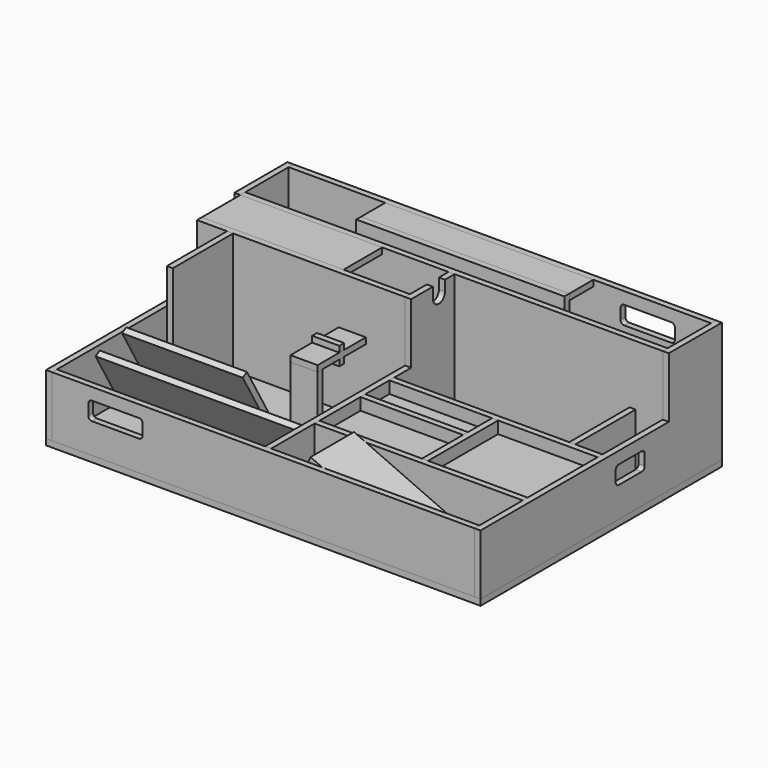
from build123d import *

# Parameters (mm, degrees)
F0_W      = 720
F0_H      = 500
F1_DEPTH  = 10
F3_DEPTH  = 10
F5_DEPTH  = 10
F6_W      = 700
F6_H      = 100
F7_DEPTH  = 10
F8_W      = 700
F8_H      = 200
F9_DEPTH  = 10
F11_DEPTH = 10
F12_W     = 345
F12_H     = 50
F13_DEPTH = 10
F14_W     = 345
F14_H     = 200
F15_DEPTH = 10
F16_W     = 235
F16_H     = 80
F17_DEPTH = 10
F19_DEPTH = 10
F21_DEPTH = 10
F22_W     = 10
F22_H     = 100
F23_DEPTH = 345
F24_W     = 10
F24_H     = 100
F25_DEPTH = 125
F26_W     = 145
F26_H     = 10
F27_DEPTH = 170
F28_W     = 145
F28_H     = 100
F29_DEPTH = 10
F30_W     = 170
F30_H     = 10
F31_DEPTH = 20
F32_W     = 145
F32_H     = 10
F33_DEPTH = 165
F35_DEPTH = 125
F36_W     = 45
F36_H     = 10
F37_DEPTH = 100
F38_W     = 45
F38_H     = 110
F39_DEPTH = 10
F40_W     = 45
F40_H     = 10
F41_DEPTH = 10
F42_START = -10
F42_DEPTH = 10
F44_DEPTH = 90
F46_DEPTH = 345
F47_W     = 200
F47_H     = 170
F48_DEPTH = 10


with BuildPart() as f1:
    # F0 (on Top) → F1 (new body)
    with BuildSketch(Plane.XY):
        Rectangle(F0_W, F0_H)
    extrude(amount=F1_DEPTH)


with BuildPart() as f3:
    # F2 (on face) → F3 (new body)
    with BuildSketch(Plane(origin=(-360, 0, 0), x_dir=(0, -1, 0), z_dir=(-1, 0, 0))):
        Polygon((-250, 110), (-250, 10), (250, 10), (250, 110), (-140, 110), (-140, 210), (-250, 210), align=None)
        with BuildLine():
            Line((-36, 60), (-84, 60))
            ThreePointArc((-84, 60), (-88.2426406871, 61.7573593129), (-90, 66))
            Line((-90, 66), (-90, 84))
            ThreePointArc((-90, 84), (-88.2426406871, 88.2426406871), (-84, 90))
            Line((-84, 90), (-36, 90))
            ThreePointArc((-36, 90), (-31.7573593129, 88.2426406871), (-30, 84))
            Line((-30, 84), (-30, 66))
            ThreePointArc((-30, 66), (-31.7573593129, 61.7573593129), (-36, 60))
        make_face(mode=Mode.SUBTRACT)
    extrude(amount=-F3_DEPTH)


with BuildPart() as f5:
    # F4 (on face) → F5 (new body)
    with BuildSketch(Plane.YZ.offset(360)):
        Polygon((-250, 10), (250, 10), (250, 210), (140, 210), (140, 110), (-250, 110), align=None)
        with BuildLine():
            ThreePointArc((90, 66), (88.2426406871, 61.7573593129), (84, 60))
            Line((84, 60), (36, 60))
            ThreePointArc((36, 60), (31.7573593129, 61.7573593129), (30, 66))
            Line((30, 66), (30, 84))
            ThreePointArc((30, 84), (31.7573593129, 88.2426406871), (36, 90))
            Line((36, 90), (84, 90))
            ThreePointArc((84, 90), (88.2426406871, 88.2426406871), (90, 84))
            Line((90, 84), (90, 66))
        make_face(mode=Mode.SUBTRACT)
    extrude(amount=-F5_DEPTH)


with BuildPart() as f7:
    # F6 (on face) → F7 (new body)
    with BuildSketch(Plane.XZ.offset(250)):
        with Locations((0, 60)):
            Rectangle(F6_W, F6_H)
        with BuildLine():
            ThreePointArc((-290, 84), (-288.2426406871, 88.2426406871), (-284, 90))
            Line((-284, 90), (-206, 90))
            ThreePointArc((-206, 90), (-201.7573593129, 88.2426406871), (-200, 84))
            Line((-200, 84), (-200, 66))
            ThreePointArc((-200, 66), (-201.7573593129, 61.7573593129), (-206, 60))
            Line((-206, 60), (-284, 60))
            ThreePointArc((-284, 60), (-288.2426406871, 61.7573593129), (-290, 66))
            Line((-290, 66), (-290, 84))
        make_face(mode=Mode.SUBTRACT)
    extrude(amount=-F7_DEPTH)


with BuildPart() as f9:
    # F8 (on face) → F9 (new body)
    with BuildSketch(Plane(origin=(0, 250, 0), x_dir=(-1, 0, 0), z_dir=(0, 1, 0))):
        with Locations((0, 110)):
            Rectangle(F8_W, F8_H)
        with BuildLine():
            Line((39, 90), (-39, 90))
            ThreePointArc((-39, 90), (-43.2426406871, 91.7573593129), (-45, 96))
            Line((-45, 96), (-45, 104))
            ThreePointArc((-45, 104), (-43.2426406871, 108.2426406871), (-39, 110))
            Line((-39, 110), (39, 110))
            ThreePointArc((39, 110), (43.2426406871, 108.2426406871), (45, 104))
            Line((45, 104), (45, 96))
            ThreePointArc((45, 96), (43.2426406871, 91.7573593129), (39, 90))
        make_face(mode=Mode.SUBTRACT)
        with BuildLine():
            ThreePointArc((-290, 184), (-288.2426406871, 188.2426406871), (-284, 190))
            Line((-284, 190), (-206, 190))
            ThreePointArc((-206, 190), (-201.7573593129, 188.2426406871), (-200, 184))
            Line((-200, 184), (-200, 166))
            ThreePointArc((-200, 166), (-201.7573593129, 161.7573593129), (-206, 160))
            Line((-206, 160), (-284, 160))
            ThreePointArc((-284, 160), (-288.2426406871, 161.7573593129), (-290, 166))
            Line((-290, 166), (-290, 184))
        make_face(mode=Mode.SUBTRACT)
    extrude(amount=-F9_DEPTH)


with BuildPart() as f11:
    # F10 (on face) → F11 (new body)
    with BuildSketch(Plane.XZ.offset(-140)):
        Polygon((-350, 210), (-350, 10), (350, 10), (350, 110), (350, 210), align=None)
    extrude(amount=-F11_DEPTH)


with BuildPart() as f13:
    # F12 (on face) → F13 (new body)
    with BuildSketch(Plane.XY.offset(210)):
        with Locations((-17.5, 215)):
            Rectangle(F12_W, F12_H)
    extrude(amount=-F13_DEPTH)


with BuildPart() as f15:
    # F14 (on face) → F15 (new body)
    with BuildSketch(Plane.XZ.offset(-190)):
        with Locations((-17.5, 110)):
            Rectangle(F14_W, F14_H)
    extrude(amount=F15_DEPTH)


with BuildPart() as f17:
    # F16 (on face) → F17 (new body)
    with BuildSketch(Plane.XY.offset(210)):
        with Locations((-232.5, 100)):
            Rectangle(F16_W, F16_H)
    extrude(amount=-F17_DEPTH)


with BuildPart() as f19:
    # F18 (on face) → F19 (new body)
    with BuildSketch(Plane.XZ.offset(-60)):
        Polygon((-5, 210), (-350, 210), (-350, 170), (-330, 145), (-300, 145), (-300, 60), (-350, 60), (-350, 10), (-5, 10), align=None)
    extrude(amount=F19_DEPTH)


with BuildPart() as f21:
    # F20 (on face) → F21 (new body)
    with BuildSketch(Plane.YZ.offset(-5)):
        with BuildLine():
            Line((60, 210), (50, 210))
            Line((50, 210), (50, 110))
            Line((50, 110), (-240, 110))
            Line((-240, 110), (-240, 10))
            Line((-240, 10), (50, 10))
            Line((50, 10), (140, 10))
            Line((140, 10), (140, 110))
            Line((140, 110), (140, 210))
            Line((140, 210), (120, 210))
            Line((120, 210), (120, 192.5))
            ThreePointArc((120, 192.5), (107.5, 180), (95, 192.5))
            Line((95, 192.5), (95, 210))
            Line((95, 210), (60, 210))
        make_face()
    extrude(amount=F21_DEPTH)


with BuildPart() as f23:
    # F22 (on face) → F23 (new body, through all)
    with BuildSketch(Plane.YZ.offset(5)):
        with Locations((10, 60)):
            Rectangle(F22_W, F22_H)
    extrude(amount=F23_DEPTH)


with BuildPart() as f23b:
    # F22 (on face) → F23, piece 2 (new body, through all)
    with BuildSketch(Plane.YZ.offset(5)):
        with Locations((-145, 60)):
            Rectangle(F22_W, F22_H)
    extrude(amount=F23_DEPTH)


with BuildPart() as f25:
    # F24 (on face) → F25 (new body, through all)
    with BuildSketch(Plane.XZ.offset(-140)):
        with Locations((300, 60)):
            Rectangle(F24_W, F24_H)
    extrude(amount=F25_DEPTH)


with BuildPart() as f27:
    # F26 (on face) → F27 (new body)
    with BuildSketch(Plane.YZ.offset(5)):
        with Locations((-67.5, 85)):
            Rectangle(F26_W, F26_H)
    extrude(amount=F27_DEPTH)


with BuildPart() as f29:
    # F28 (on face) → F29 (new body)
    with BuildSketch(Plane.YZ.offset(175)):
        with Locations((-67.5, 60)):
            Rectangle(F28_W, F28_H)
    extrude(amount=F29_DEPTH)


with BuildPart() as f31:
    # F30 (on face) → F31 (new body, through all)
    with BuildSketch(Plane.XY.offset(90)):
        with Locations((90, -50)):
            Rectangle(F30_W, F30_H)
    extrude(amount=F31_DEPTH)


with BuildPart() as f33:
    # F32 (on face) → F33 (new body, through all)
    with BuildSketch(Plane.YZ.offset(185)):
        with Locations((-67.5, 85)):
            Rectangle(F32_W, F32_H)
    extrude(amount=F33_DEPTH)


with BuildPart() as f35:
    # F34 (on face) → F35 (new body)
    with BuildSketch(Plane.XZ.offset(-50)):
        Polygon((-300, 145), (-300, 60), (-300, 10), (-290, 10), (-290, 210), (-300, 210), align=None)
    extrude(amount=F35_DEPTH)


with BuildPart() as f37:
    # F36 (on face) → F37 (new body)
    with BuildSketch(Plane.XZ.offset(-50)):
        with Locations((-92.5, 125)):
            Rectangle(F36_W, F36_H)
    extrude(amount=F37_DEPTH)


with BuildPart() as f39:
    # F38 (on face) → F39 (new body)
    with BuildSketch(Plane.XZ.offset(50)):
        with Locations((-92.5, 65)):
            Rectangle(F38_W, F38_H)
    extrude(amount=-F39_DEPTH)


with BuildPart() as f41:
    # F40 (on face) → F41 (new body)
    with BuildSketch(Plane.XY.offset(130)):
        with Locations((-92.5, 0)):
            Rectangle(F40_W, F40_H)
    extrude(amount=F41_DEPTH)


with BuildPart() as f42:
    # F40 (on face) → F42 (new body)
    with BuildSketch(Plane.XY.offset(130).offset(F42_START)):
        with Locations((-92.5, 0)):
            Rectangle(F40_W, F40_H)
    extrude(amount=-F42_DEPTH)


with BuildPart() as f44:
    # F43 (on face) → F44 (new body, through all)
    with BuildSketch(Plane.XZ.offset(150)):
        Polygon((66.1813628776, 109.6504775536), (290, 10), (294.0673664308, 19.1354545764), (70.2487293083, 118.78593213), align=None)
    extrude(amount=F44_DEPTH)


with BuildPart() as f46:
    # F45 (on face) → F46 (new body, through all)
    with BuildSketch(Plane(origin=(-5, 0, 0), x_dir=(0, -1, 0), z_dir=(-1, 0, 0))):
        Polygon((101.3397459622, 15), (110, 10), (160, 96.6025403784), (151.3397459622, 101.6025403784), align=None)
    extrude(amount=F46_DEPTH)


with BuildPart() as f48:
    # F47 (on face) → F48 (new body)
    with BuildSketch(Plane(origin=(0, -69.5096189432, -40.1313972081), x_dir=(-1, 0, 0), z_dir=(0, 0.8660254038, 0.5))):
        with Locations((185, 148.6602540378)):
            Rectangle(F47_W, F47_H)
    extrude(amount=F48_DEPTH)


with BuildPart() as f50_1:
    # F50: copy of F3
    add(f3.part.moved(Location((700, 0, 0))))


with BuildPart() as f50_1_1:
    # F51: moved
    add(f50_1.part.moved(Location((10, 0, 0))))


solid = Compound([f1.part, f3.part, f7.part, f9.part, f11.part, f13.part, f15.part, f17.part, f19.part, f21.part, f23.part, f23b.part, f25.part, f27.part, f29.part, f31.part, f33.part, f35.part, f37.part, f39.part, f41.part, f42.part, f44.part, f46.part, f48.part, f50_1_1.part])
